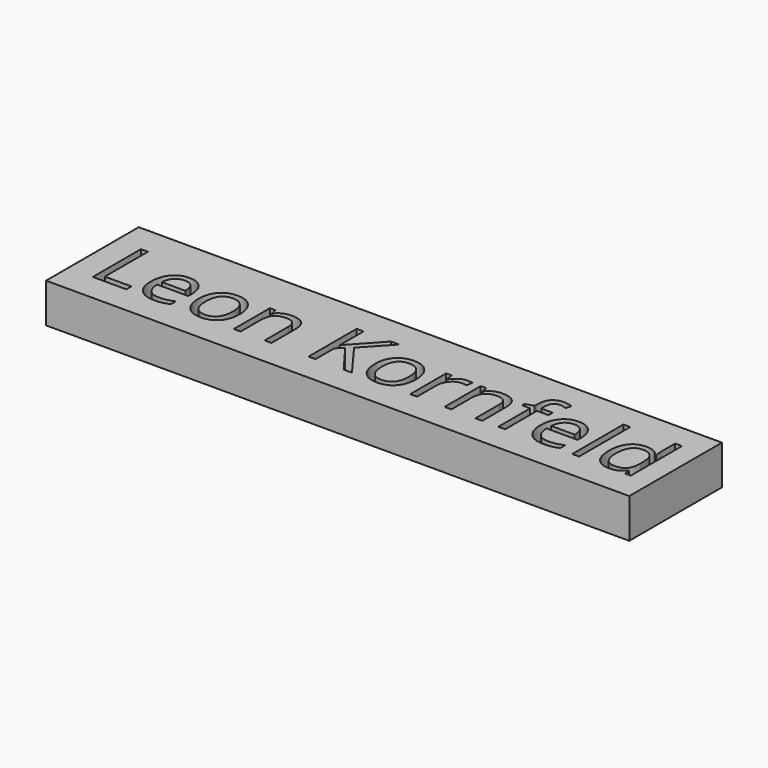
from build123d import *

# Parameters (mm, degrees)
F0_W         = 93.98
F0_H         = 18.6602950151
F1_DEPTH     = 6.35
F2_TEXT_SIZE = 13.5884024743
F3_DEPTH     = 16.764


# Not quite as in the source:
# - Text() gives the source's letters only with a copy of the font that has no kerning and outlines rounded to 1/6400 em; it was checked with that copy


with BuildPart() as f1:
    # F0 (on Top) → F1 (new body)
    with BuildSketch(Plane.XY):
        Rectangle(F0_W, F0_H)
    extrude(amount=F1_DEPTH)

    # F2 (on Top) → F3 (cut)
    with BuildSketch(Plane.XY):
        with Locations((-44.3652127803, -4.8715729289)):
            Text('Leon Kornfeld', F2_TEXT_SIZE, font='Open Sans', text_align=(TextAlign.LEFT, TextAlign.BOTTOM))
    extrude(amount=F3_DEPTH, mode=Mode.SUBTRACT)


solid = f1.part
